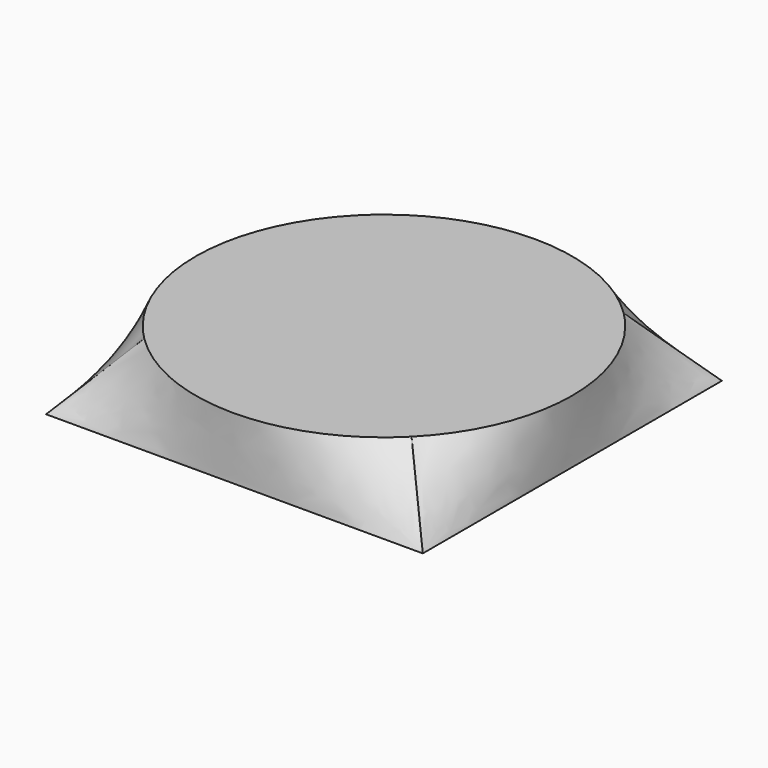
from build123d import *

# Parameters (mm, degrees)
F2_W = 151.9237607718
F2_H = 150.7853120565


# Not quite as in the source:
# - the arcs of a loft's sections are written as splines that run evenly, so that the points pair up as in the source's solid


with BuildPart() as f3:
    # F1 (on offset) → F3 section 0
    with BuildSketch(Plane.XY.offset(25.4)):
        with BuildLine():
            add(Edge.make_bspline(
                [(-53.9234495618, 53.5193713481), (-57.4262842254, 49.9900898272), (-60.5814369798, 46.1159050039), (-66.0754369985, 37.8262319869), (-68.4141484128, 33.4109487717), (-72.1853477833, 24.2087332645), (-73.6177424893, 19.4220285153), (-75.5212161348, 9.6609064991), (-75.9922480073, 4.686730595), (-75.9548465031, -5.2581834851), (-75.4464140513, -10.2286757536), (-73.4695747162, -19.9752044268), (-72.0012167141, -24.7509998294), (-68.1609083751, -33.9245894647), (-65.7890529974, -38.3221568623), (-60.2328565503, -46.5702715545), (-57.0486528689, -50.4206148982), (-53.5193713481, -53.9234495618)],
                knots=[0, 0, 0, 0, 0.125, 0.125, 0.25, 0.25, 0.375, 0.375, 0.5, 0.5, 0.625, 0.625, 0.75, 0.75, 0.875, 0.875, 1, 1, 1, 1], degree=3))
            add(Edge.make_bspline(
                [(-53.5193713481, -53.9234495618), (-49.9900898272, -57.4262842254), (-46.1159050039, -60.5814369798), (-37.8262319869, -66.0754369985), (-33.4109487717, -68.4141484128), (-24.2087332645, -72.1853477833), (-19.4220285153, -73.6177424893), (-9.6609064991, -75.5212161348), (-4.686730595, -75.9922480073), (5.2581834851, -75.9548465031), (10.2286757536, -75.4464140513), (19.9752044268, -73.4695747162), (24.7509998294, -72.0012167141), (33.9245894647, -68.1609083751), (38.3221568623, -65.7890529974), (46.5702715545, -60.2328565503), (50.4206148982, -57.0486528689), (53.9234495618, -53.5193713481)],
                knots=[0, 0, 0, 0, 0.125, 0.125, 0.25, 0.25, 0.375, 0.375, 0.5, 0.5, 0.625, 0.625, 0.75, 0.75, 0.875, 0.875, 1, 1, 1, 1], degree=3))
            add(Edge.make_bspline(
                [(53.9234495618, -53.5193713481), (57.4262842254, -49.9900898272), (60.5814369798, -46.1159050039), (66.0754369985, -37.8262319869), (68.4141484128, -33.4109487717), (72.1853477833, -24.2087332645), (73.6177424893, -19.4220285153), (75.5212161348, -9.6609064991), (75.9922480073, -4.686730595), (75.9548465031, 5.2581834851), (75.4464140513, 10.2286757536), (73.4695747162, 19.9752044268), (72.0012167141, 24.7509998294), (68.1609083751, 33.9245894647), (65.7890529974, 38.3221568623), (60.2328565503, 46.5702715545), (57.0486528689, 50.4206148982), (53.5193713481, 53.9234495618)],
                knots=[0, 0, 0, 0, 0.125, 0.125, 0.25, 0.25, 0.375, 0.375, 0.5, 0.5, 0.625, 0.625, 0.75, 0.75, 0.875, 0.875, 1, 1, 1, 1], degree=3))
            add(Edge.make_bspline(
                [(53.5193713481, 53.9234495618), (49.9900898272, 57.4262842254), (46.1159050039, 60.5814369798), (37.8262319869, 66.0754369985), (33.4109487717, 68.4141484128), (24.2087332645, 72.1853477833), (19.4220285153, 73.6177424893), (9.6609064991, 75.5212161348), (4.686730595, 75.9922480073), (-5.2581834851, 75.9548465031), (-10.2286757536, 75.4464140513), (-19.9752044268, 73.4695747162), (-24.7509998294, 72.0012167141), (-33.9245894647, 68.1609083751), (-38.3221568623, 65.7890529974), (-46.5702715545, 60.2328565503), (-50.4206148982, 57.0486528689), (-53.9234495618, 53.5193713481)],
                knots=[0, 0, 0, 0, 0.125, 0.125, 0.25, 0.25, 0.375, 0.375, 0.5, 0.5, 0.625, 0.625, 0.75, 0.75, 0.875, 0.875, 1, 1, 1, 1], degree=3))
        make_face()
    # F2 (on Top) → F3 section 1
    with BuildSketch(Plane.XY):
        Rectangle(F2_W, F2_H)
    loft(ruled=True)


solid = f3.part
